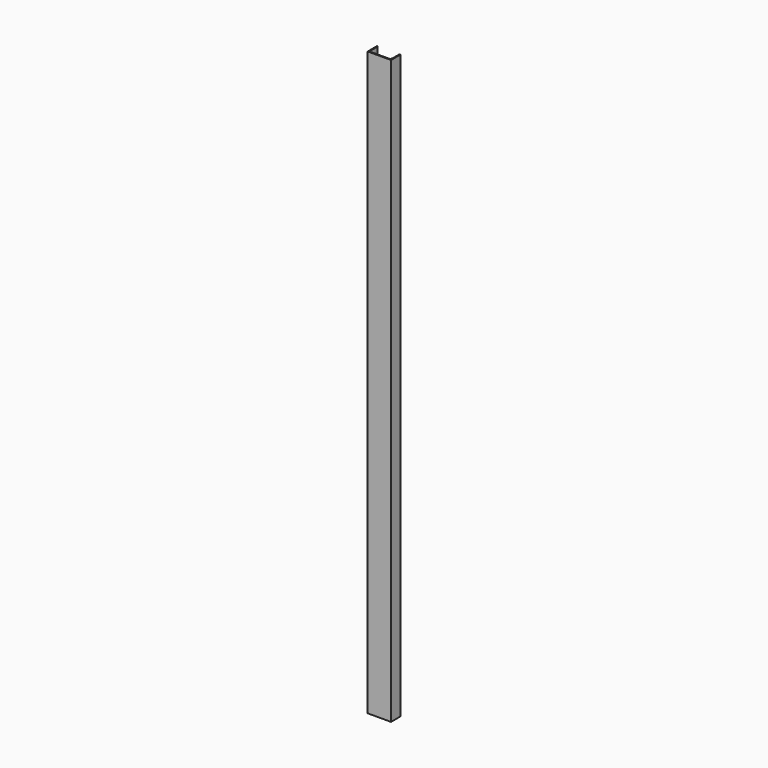
from build123d import *

# Parameters (mm, degrees)
F1_DEPTH    = 2500
F2_T1_DEPTH = 2500
F3_R        = 3.99999


# Not quite as in the source:
# - a fillet or chamfer that OpenCascade refuses, or shapes differently, is made with other operations: its cross-section is extruded or revolved along the edge and cut away or added
# - a fillet or chamfer is up to 0.001 mm smaller than in the source, because OpenCascade refuses the exact size


with BuildPart() as f1:
    # F0 (on Top) → F1 (new body)
    with BuildSketch(Plane.XY):
        Polygon((-50, -25), (50, -25), (50, 25), (46, 25), (46, -21), (-46, -21), (-46, 25), (-50, 25), align=None)
    extrude(amount=F1_DEPTH)

    # F2: fillet of radius 10 on 2 edges, made by hand

    # F2_s2 → F2_t1 (join)
    with BuildSketch(Plane.XY):
        with BuildLine():
            add(Edge.make_bspline(
                [(46, -11), (46, -21), (36, -21)],
                knots=[0, 0, 0, 1, 1, 1], degree=2, weights=[1, 1, 1]))
            Line((36, -21), (46, -21))
            Line((46, -21), (46, -11))
        make_face()
        with BuildLine():
            add(Edge.make_bspline(
                [(-36, -21), (-46, -21), (-46, -11)],
                knots=[0, 0, 0, 1, 1, 1], degree=2, weights=[1, 1, 1]))
            Line((-46, -11), (-46, -21))
            Line((-46, -21), (-36, -21))
        make_face()
    extrude(amount=F2_T1_DEPTH)

    # F3 (radius 4 in the source; OpenCascade refuses exactly that, so slightly less here)
    f3_edges = [f1.edges().sort_by_distance(p)[0] for p in [
        (-46, 25, 1250),
        (46, 25, 1250),
    ]]
    fillet(f3_edges, radius=F3_R)


solid = f1.part
